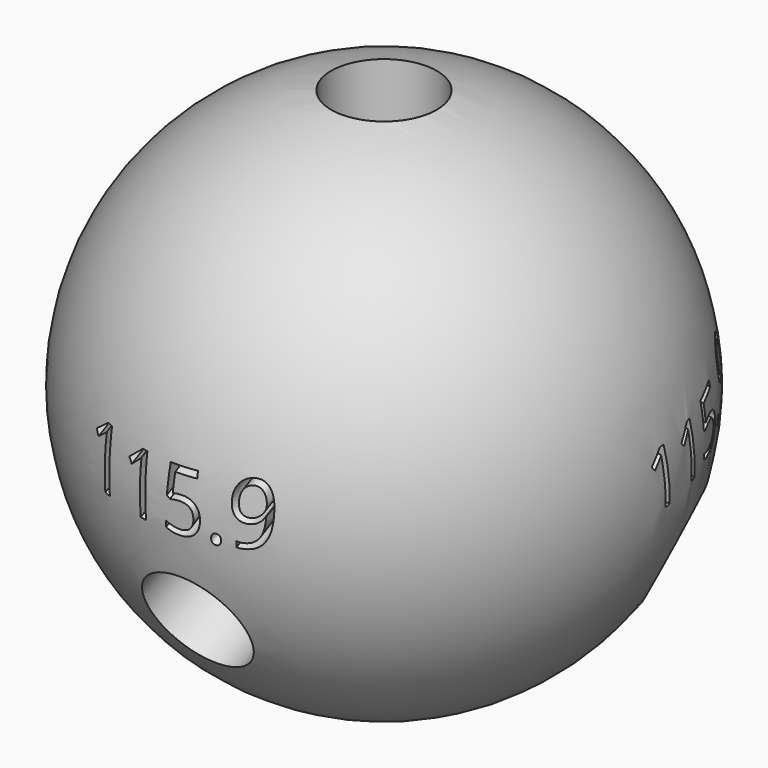
from build123d import *

# Parameters (mm, degrees)
F4_R          = 3.175
F5_DEPTH      = 25.4
F8_ANGLE      = 115.9
F10_TEXT_SIZE = 4.4808457864
F11_DEPTH     = 7.62
F12_ANGLE     = 115.4
F14_TEXT_SIZE = 4.3551120648
F15_DEPTH     = 7.62
F17_ANGLE     = 94.7
F19_ANGLE     = -105.7
F21_TEXT_SIZE = 5.0597895299
F22_DEPTH     = 7.62


# Not quite as in the source:
# - Text() gives the source's letters only with a copy of the font that has no kerning and outlines rounded to 1/6400 em; it was checked with that copy


with BuildPart() as f2:
    # F1 (on Top) → F2 (revolve)
    with BuildSketch(Plane.XY):
        with BuildLine():
            Line((0, -15.875), (0, 15.875))
            ThreePointArc((0, 15.875), (-15.875, 0), (0, -15.875))
        make_face()
    revolve(axis=Axis((0, 0, 0), (0, -1, 0)))

    # F10 (on offset) → F11 (cut)
    with BuildSketch(Plane(origin=(0, -17.1365756891, -8.3210740684), x_dir=(1, 0, 0), z_dir=(0, -0.899557779, -0.4368017884))):
        with Locations((-5.8622976067, 5.6281532161)):
            Text('115.9', F10_TEXT_SIZE, font='Open Sans', text_align=(TextAlign.LEFT, TextAlign.BOTTOM))
    extrude(amount=-F11_DEPTH, mode=Mode.SUBTRACT)

    # F14 (on offset) → F15 (cut)
    with BuildSketch(Plane(origin=(15.4800736188, 7.3504793793, -8.3210740684), x_dir=(-0.339862905, 0.9225607208, 0.1826880463), z_dir=(0.8126022897, 0.3858519359, -0.4368017884))):
        with Locations((-5.4003379009, 5.5745393038)):
            Text('115.9', F14_TEXT_SIZE, font='Open Sans', text_align=(TextAlign.LEFT, TextAlign.BOTTOM))
    extrude(amount=-F15_DEPTH, mode=Mode.SUBTRACT)

    # F21 (on offset) → F22 (cut)
    with BuildSketch(Plane(origin=(-18.2776098722, 5.1376044317, -1.5609285894), x_dir=(-0.2687123943, -0.9629470508, -0.0229483429), z_dir=(-0.9594545865, 0.2696905213, -0.0819385086))):
        with Locations((-5.084984994, 5.6783161126)):
            Text('94.7', F21_TEXT_SIZE, font='Open Sans', text_align=(TextAlign.LEFT, TextAlign.BOTTOM))
    extrude(amount=-F22_DEPTH, mode=Mode.SUBTRACT)


with BuildPart() as f5:
    # F4 (on offset) → F5 (new body)
    with BuildSketch(Plane.XY.offset(6.35)):
        Circle(F4_R)
    extrude(amount=F5_DEPTH)


with BuildPart() as f8_1:
    # F8: copy of F5
    add(f5.part.rotate(Axis((26.8236305565, 0, 0), (1, 0, 0)), F8_ANGLE))


with BuildPart() as f12_1:
    # F12: copy of F8_1
    add(f8_1.part.rotate(Axis((0, 0, 29.4045954943), (0, 0, 1)), F12_ANGLE))


with BuildPart() as f17_1:
    # F17: copy of F5
    add(f5.part.rotate(Axis((31.2481448054, 0, 0), (1, 0, 0)), F17_ANGLE))


with BuildPart() as f17_1_1:
    # F19: moved
    add(f17_1.part.rotate(Axis((0, 0, 32.354272902), (0, 0, 1)), F19_ANGLE))


with BuildPart() as f2_1:
    add(f2.part)

    # F23: cut F5, F17_1, F8_1, F12_1
    add(f5.part, mode=Mode.SUBTRACT)
    add(f17_1_1.part, mode=Mode.SUBTRACT)
    add(f8_1.part, mode=Mode.SUBTRACT)
    add(f12_1.part, mode=Mode.SUBTRACT)


solid = f2_1.part
